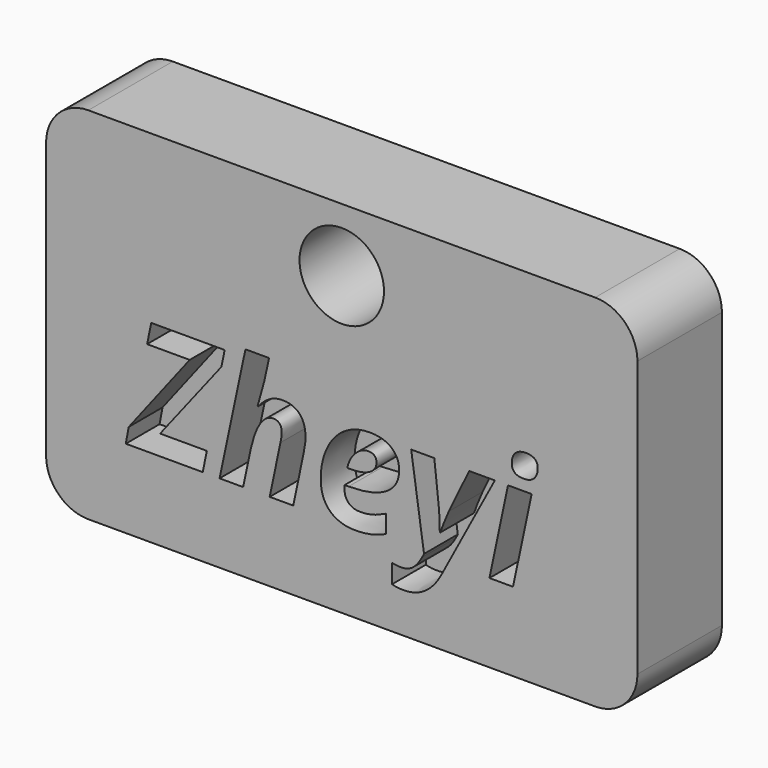
from build123d import *

# Parameters (mm, degrees)
F0_W         = 71.12
F0_H         = 43.3009530022
F1_DEPTH     = 12.7
F2_TEXT_SIZE = 19.3155893536
F3_DEPTH     = 5.08
F5_DEPTH     = 12.701
F6_R         = 5.08


# Not quite as in the source:
# - Text() gives the source's letters only with a copy of the font that has no kerning and outlines rounded to 1/6400 em; it was checked with that copy


with BuildPart() as f1:
    # F0 (on Front) → F1 (new body)
    with BuildSketch(Plane.XZ):
        Rectangle(F0_W, F0_H)
    extrude(amount=F1_DEPTH)

    # F2 (on face) → F3 (cut)
    with BuildSketch(Plane.XZ.offset(12.7)):
        with Locations((-25.4, -12.1874138805)):
            Text('Zheyi', F2_TEXT_SIZE, font='Open Sans', font_style=FontStyle.BOLDITALIC, text_align=(TextAlign.LEFT, TextAlign.BOTTOM))
    extrude(amount=-F3_DEPTH, mode=Mode.SUBTRACT)

    # F4 (on face) → F5 (cut, through all)
    with BuildSketch(Plane.XZ.offset(12.7)):
        with BuildLine():
            ThreePointArc((0, 19.1104765011), (-3.5921024484, 10.4383740527), (5.08, 14.0304765011))
            ThreePointArc((5.08, 14.0304765011), (3.5921024484, 17.6225789495), (0, 19.1104765011))
        make_face()
    extrude(amount=-F5_DEPTH, mode=Mode.SUBTRACT)

    # F6
    f6_edges = [f1.edges().sort_by_distance(p)[0] for p in [
        (35.56, -6.35, 21.650477),
        (-35.56, -6.35, 21.650477),
        (35.56, -6.35, -21.650477),
        (-35.56, -6.35, -21.650477),
    ]]
    fillet(f6_edges, radius=F6_R)


solid = f1.part
